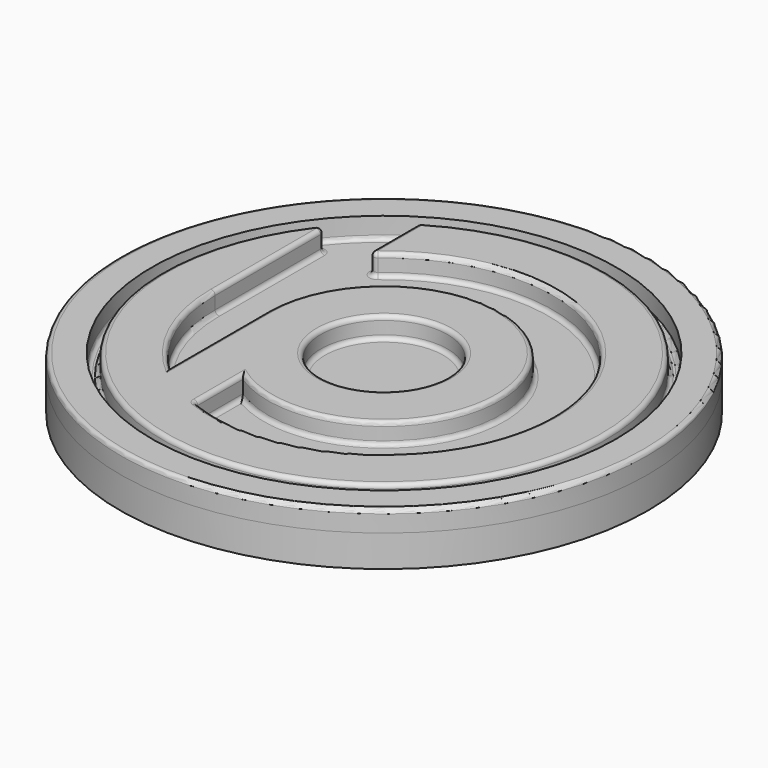
from build123d import *

# Parameters (mm, degrees)
F0_R     = 12.5
F0_R_2   = 11
F0_R_3   = 3
F1_DEPTH = 1.5
F2_DEPTH = 1
F3_R     = 0.2


with BuildPart() as f1:
    # F0 (on Top) → F1 (new body)
    with BuildSketch(Plane.XY):
        with Locations((-248.9948847865, 13.3405361525)):
            Circle(F0_R)
        with Locations((-248.9948847865, 13.3405361525)):
            Circle(F0_R_2, mode=Mode.SUBTRACT)
        with Locations((-248.9948847865, 13.3405361525)):
            Circle(F0_R_2)
        with BuildLine():
            ThreePointArc((-254.4948847865, 13.3405361525), (-244.1601148851, 15.9625582729), (-251.9948847865, 8.7307639238))
            Line((-251.9948847865, 8.7307639238), (-251.9948847865, 5.9243376654))
            ThreePointArc((-251.9948847865, 5.9243376654), (-241.1340890301, 14.8264332134), (-254.4948847865, 19.1500111718))
            Line((-254.4948847865, 19.1500111718), (-254.4948847865, 22.2848080625))
            ThreePointArc((-254.4948847865, 22.2848080625), (-242.1603264724, 5.3694124769), (-256.9948847865, 20.1412714069))
            Line((-256.9948847865, 20.1412714069), (-256.9948847865, 13.3405361525))
            ThreePointArc((-256.9948847865, 13.3405361525), (-256.3433540149, 10.1782584923), (-254.4948847865, 7.5310611332))
            Line((-254.4948847865, 7.5310611332), (-254.4948847865, 13.3405361525))
        make_face(mode=Mode.SUBTRACT)
        with BuildLine():
            Line((-251.9948847865, 5.9243376654), (-251.9948847865, 8.7307639238))
            ThreePointArc((-251.9948847865, 8.7307639238), (-244.1601148851, 15.9625582729), (-254.4948847865, 13.3405361525))
            Line((-254.4948847865, 13.3405361525), (-254.4948847865, 7.5310611332))
            ThreePointArc((-254.4948847865, 7.5310611332), (-256.3433540149, 10.1782584923), (-256.9948847865, 13.3405361525))
            Line((-256.9948847865, 13.3405361525), (-256.9948847865, 20.1412714069))
            ThreePointArc((-256.9948847865, 20.1412714069), (-242.1603264724, 5.3694124769), (-254.4948847865, 22.2848080625))
            Line((-254.4948847865, 22.2848080625), (-254.4948847865, 19.1500111718))
            ThreePointArc((-254.4948847865, 19.1500111718), (-241.1340890301, 14.8264332134), (-251.9948847865, 5.9243376654))
        make_face()
        with Locations((-248.9948847865, 13.3405361525)):
            Circle(F0_R_3, mode=Mode.SUBTRACT)
        with Locations((-248.9948847865, 13.3405361525)):
            Circle(F0_R_3)
    extrude(amount=-F1_DEPTH)

    # F0 (on Top) → F2 (join)
    with BuildSketch(Plane.XY):
        with Locations((-248.9948847865, 13.3405361525)):
            Circle(F0_R)
        with Locations((-248.9948847865, 13.3405361525)):
            Circle(F0_R_2, mode=Mode.SUBTRACT)
        with BuildLine():
            Line((-251.9948847865, 5.9243376654), (-251.9948847865, 8.7307639238))
            ThreePointArc((-251.9948847865, 8.7307639238), (-244.1601148851, 15.9625582729), (-254.4948847865, 13.3405361525))
            Line((-254.4948847865, 13.3405361525), (-254.4948847865, 7.5310611332))
            ThreePointArc((-254.4948847865, 7.5310611332), (-256.3433540149, 10.1782584923), (-256.9948847865, 13.3405361525))
            Line((-256.9948847865, 13.3405361525), (-256.9948847865, 20.1412714069))
            ThreePointArc((-256.9948847865, 20.1412714069), (-242.1603264724, 5.3694124769), (-254.4948847865, 22.2848080625))
            Line((-254.4948847865, 22.2848080625), (-254.4948847865, 19.1500111718))
            ThreePointArc((-254.4948847865, 19.1500111718), (-241.1340890301, 14.8264332134), (-251.9948847865, 5.9243376654))
        make_face()
        with Locations((-248.9948847865, 13.3405361525)):
            Circle(F0_R_3, mode=Mode.SUBTRACT)
    extrude(amount=F2_DEPTH)

    # F3
    f3_edges = [f1.edges().sort_by_distance(p)[0] for p in [
        (-261.494885, 13.340536, 1),
        (-256.994885, 16.740904, 1),
        (-256.343354, 10.178258, 1),
        (-254.494885, 20.71741, 1),
        (-254.494885, 10.435799, 1),
        (-251.994885, 7.327551, 1),
        (-251.994885, 13.340536, 0),
        (-241.134089, 14.826433, 0),
        (-244.160115, 15.962558, 0),
        (-254.494885, 10.435799, 0),
        (-254.494885, 20.71741, 0),
        (-259.994885, 13.340536, 0),
        (-242.160326, 5.369412, 0),
        (-251.994885, 13.340536, 1),
        (-241.134089, 14.826433, 1),
        (-251.994885, 7.327551, 0),
        (-251.994885, 5.924338, 0.5),
        (-254.494885, 19.150011, 0.5),
        (-254.494885, 22.284808, 0.5),
        (-256.994885, 20.141271, 0.5),
        (-244.160115, 15.962558, 1),
        (-242.160326, 5.369412, 1),
        (-256.343354, 10.178258, 0),
        (-256.994885, 16.740904, 0),
    ]]
    fillet(f3_edges, radius=F3_R)


solid = f1.part
